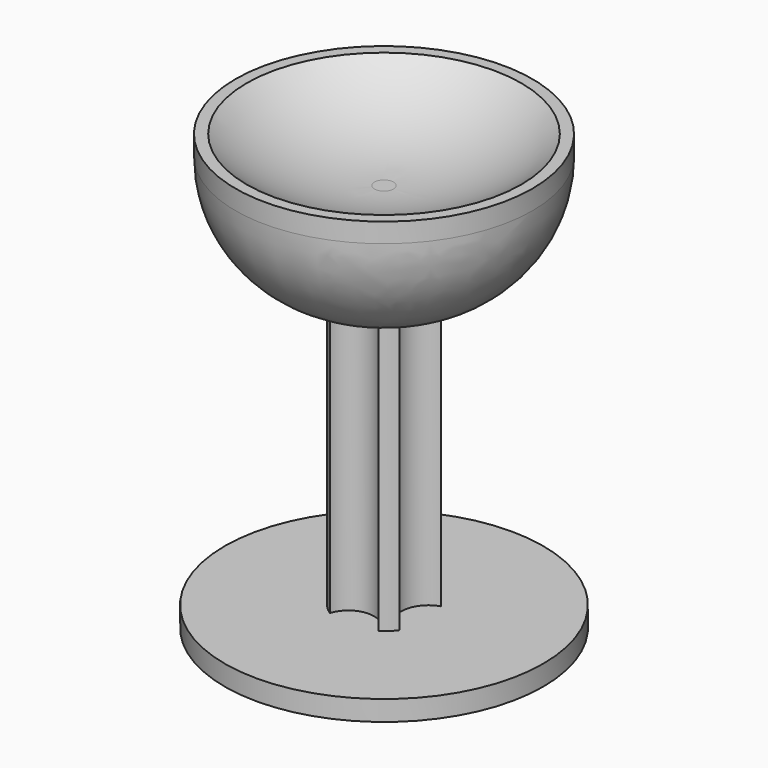
from build123d import *

# Parameters (mm, degrees)
F0_R         = 4
F1_DEPTH     = 0.508
F3_DEPTH     = 6.858
F4_R         = 3.7280143699
F5_DEPTH     = 3.556
F6_S4_R      = 1.1174755471
F6_T5_DEPTH  = 7
F6_S9_R      = 0.6824583231
F6_T10_DEPTH = 7
F6_S14_R     = 0.6735395425
F6_T15_DEPTH = 7
F6_S19_R     = 0.7128054748
F6_T20_DEPTH = 7
F6_S24_R     = 0.6367238251
F6_T25_DEPTH = 7
F7_R         = 3.448614385
F8_DEPTH     = 1.143


# Not quite as in the source:
# - a fillet or chamfer that OpenCascade refuses, or shapes differently, is made with other operations: its cross-section is extruded or revolved along the edge and cut away or added
# - after a boolean that leaves OpenCascade's solid faulty, fix() repairs it


with BuildPart() as f1:
    # F0 (on Top) → F1 (new body)
    with BuildSketch(Plane.XY):
        Circle(F0_R)
    extrude(amount=F1_DEPTH)

    # F2 (on face) → F3 (join)
    with BuildSketch(Plane.XY.offset(0.508)):
        with BuildLine():
            ThreePointArc((0.9090820105, -0.6498626752), (0.435017224, 0), (0.9090820105, 0.6498626752))
            ThreePointArc((0.9090820105, 0.6498626752), (0.786858404, 0.7934768115), (0.6422255841, 0.9144932463))
            ThreePointArc((0.6422255841, 0.9144932463), (0, 0.4439360046), (-0.6422255841, 0.9144932463))
            ThreePointArc((-0.6422255841, 0.9144932463), (-0.775437459, 0.8046417498), (-0.8901365032, 0.6755801981))
            ThreePointArc((-0.8901365032, 0.6755801981), (-0.5386231652, 0.4159586096), (-0.4046700723, 0))
            ThreePointArc((-0.4046700723, 0), (-0.5386231652, -0.4159586096), (-0.8901365032, -0.6755801981))
            ThreePointArc((-0.8901365032, -0.6755801981), (-0.7614591966, -0.8178823205), (-0.6103373986, -0.9360768442))
            ThreePointArc((-0.6103373986, -0.9360768442), (0, -0.480751722), (0.6103373986, -0.9360768442))
            ThreePointArc((0.6103373986, -0.9360768442), (0.7730708071, -0.8069158107), (0.9090820105, -0.6498626752))
        make_face()
    extrude(amount=F3_DEPTH)

    # F4 (on face) → F5 (join)
    with BuildSketch(Plane.XY.offset(7.366)):
        Circle(F4_R)
    extrude(amount=F5_DEPTH)

    # F6: fillet of radius 3.0660512242 on 1 edges, made by hand


with BuildPart() as f6_tool1:
    # F6_s2 → F6_t3 (revolve)
    with BuildSketch(Plane.XZ):
        with BuildLine():
            ThreePointArc((3.7280143699, 10.4320512242), (2.8299887577, 8.2640256121), (0.6619631456, 7.366))
            Line((0.6619631456, 7.366), (3.7280143699, 7.366))
            Line((3.7280143699, 7.366), (3.7280143699, 10.4320512242))
        make_face()
    revolve(axis=Axis((0, 0, 7.366), (0, 0, 1)))

    # F6_s4 → F6_t5 (cut, symmetric)
    with BuildSketch(Plane.XY.offset(8.9)):
        Circle(F6_S4_R)
    extrude(amount=F6_T5_DEPTH, both=True, mode=Mode.SUBTRACT)


with BuildPart() as f6_tool6:
    # F6_s7 → F6_t8 (revolve)
    with BuildSketch(Plane.XZ):
        with BuildLine():
            ThreePointArc((3.7280143699, 10.4320512242), (2.8299887577, 8.2640256121), (0.6619631456, 7.366))
            Line((0.6619631456, 7.366), (3.7280143699, 7.366))
            Line((3.7280143699, 7.366), (3.7280143699, 10.4320512242))
        make_face()
    revolve(axis=Axis((0, 0, 7.366), (0, 0, 1)))

    # F6_s9 → F6_t10 (intersect, symmetric)
    with BuildSketch(Plane.XY.offset(8.9)):
        with Locations((1.1174755471, 0)):
            Circle(F6_S9_R)
    extrude(amount=F6_T10_DEPTH, both=True, mode=Mode.INTERSECT)


with BuildPart() as f6_tool11:
    # F6_s12 → F6_t13 (revolve)
    with BuildSketch(Plane.XZ):
        with BuildLine():
            ThreePointArc((3.7280143699, 10.4320512242), (2.8299887577, 8.2640256121), (0.6619631456, 7.366))
            Line((0.6619631456, 7.366), (3.7280143699, 7.366))
            Line((3.7280143699, 7.366), (3.7280143699, 10.4320512242))
        make_face()
    revolve(axis=Axis((0, 0, 7.366), (0, 0, 1)))

    # F6_s14 → F6_t15 (intersect, symmetric)
    with BuildSketch(Plane.XY.offset(8.9)):
        with Locations((0, 1.1174755471)):
            Circle(F6_S14_R)
    extrude(amount=F6_T15_DEPTH, both=True, mode=Mode.INTERSECT)


with BuildPart() as f6_tool16:
    # F6_s17 → F6_t18 (revolve)
    with BuildSketch(Plane.XZ):
        with BuildLine():
            ThreePointArc((3.7280143699, 10.4320512242), (2.8299887577, 8.2640256121), (0.6619631456, 7.366))
            Line((0.6619631456, 7.366), (3.7280143699, 7.366))
            Line((3.7280143699, 7.366), (3.7280143699, 10.4320512242))
        make_face()
    revolve(axis=Axis((0, 0, 7.366), (0, 0, 1)))

    # F6_s19 → F6_t20 (intersect, symmetric)
    with BuildSketch(Plane.XY.offset(8.9)):
        with Locations((-1.1174755471, 0)):
            Circle(F6_S19_R)
    extrude(amount=F6_T20_DEPTH, both=True, mode=Mode.INTERSECT)


with BuildPart() as f6_tool21:
    # F6_s22 → F6_t23 (revolve)
    with BuildSketch(Plane.XZ):
        with BuildLine():
            ThreePointArc((3.7280143699, 10.4320512242), (2.8299887577, 8.2640256121), (0.6619631456, 7.366))
            Line((0.6619631456, 7.366), (3.7280143699, 7.366))
            Line((3.7280143699, 7.366), (3.7280143699, 10.4320512242))
        make_face()
    revolve(axis=Axis((0, 0, 7.366), (0, 0, 1)))

    # F6_s24 → F6_t25 (intersect, symmetric)
    with BuildSketch(Plane.XY.offset(8.9)):
        with Locations((0, -1.1174755471)):
            Circle(F6_S24_R)
    extrude(amount=F6_T25_DEPTH, both=True, mode=Mode.INTERSECT)


with BuildPart() as f1_1:
    add(f1.part)

    # F6_t26: cut F6_tool1, F6_tool6, F6_tool11, F6_tool16, F6_tool21
    add([f6_tool1.part, f6_tool6.part, f6_tool11.part, f6_tool16.part, f6_tool21.part], mode=Mode.SUBTRACT)

    # F7 (on face) → F8 (cut)
    with BuildSketch(Plane.XY.offset(10.922)):
        Circle(F7_R)
    extrude(amount=-F8_DEPTH, mode=Mode.SUBTRACT)

    add(f1_1.part.fix(), mode=Mode.REPLACE)

    # F9: fillet of radius 5.08 on 1 edges, made by hand

    # F9_s1 → F9_t2 (revolve)
    with BuildSketch(Plane.XZ):
        with BuildLine():
            ThreePointArc((3.448614385, 10.922), (1.9421351203, 10.0732733049), (0.2382513214, 9.779))
            Line((0.2382513214, 9.779), (0.2382513214, 9.6774))
            Line((0.2382513214, 9.6774), (3.448614385, 9.6774))
            Line((3.448614385, 9.6774), (3.550214385, 9.779))
            ThreePointArc((3.550214385, 9.779), (3.550214385, 10.3505), (3.5128216463, 10.84326))
            Line((3.5128216463, 10.84326), (3.448614385, 10.922))
        make_face()
    revolve(axis=Axis((0, 0, 9.779), (0, 0, 1)))


solid = f1_1.part
